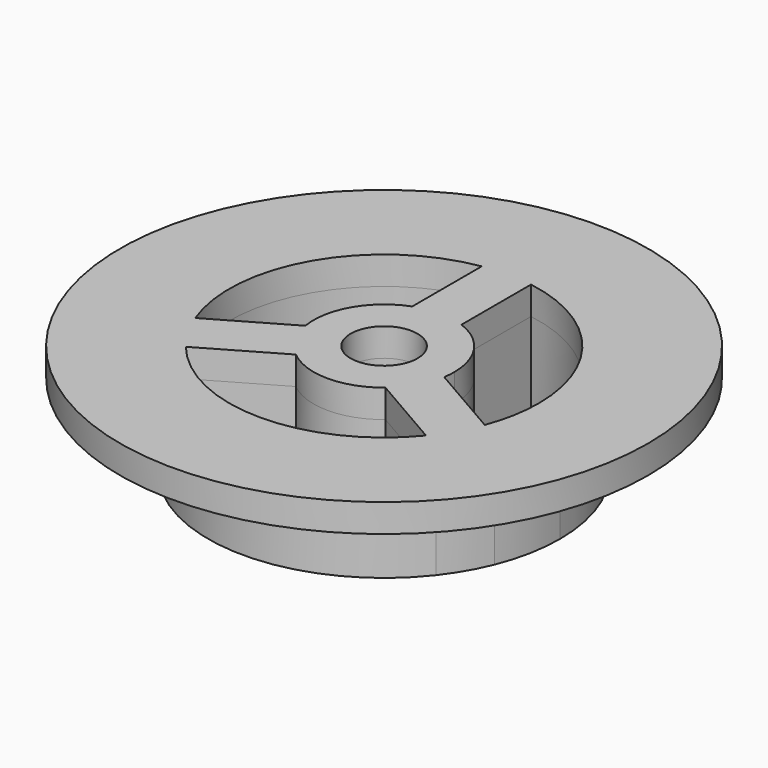
from build123d import *
from build123d import SkipClean  # not in build123d's __all__

# Parameters (mm, degrees)
F0_R     = 37.5
F0_R_2   = 4.75
F1_DEPTH = 4
F2_DEPTH = 12


with BuildPart() as f1:
    # F0 (on Top) → F1 (new body)
    with BuildSketch(Plane.XY):
        Circle(F0_R)
        with BuildLine():
            ThreePointArc((3.5, 24.753787589), (18.8745860882, 16.3935963108), (25, 0))
            ThreePointArc((25, 0), (24.5426691937, -4.7599778204), (23.1874088919, -9.3458048812))
            ThreePointArc((23.1874088919, -9.3458048812), (21.6506350946, -12.5), (19.6874088919, -15.4079827077))
            ThreePointArc((19.6874088919, -15.4079827077), (0, -25), (-19.6874088919, -15.4079827077))
            ThreePointArc((-19.6874088919, -15.4079827077), (-21.6506350946, -12.5), (-23.1874088919, -9.3458048812))
            ThreePointArc((-23.1874088919, -9.3458048812), (-21.6506350946, 12.5), (-3.5, 24.753787589))
            ThreePointArc((-3.5, 24.753787589), (0, 25), (3.5, 24.753787589))
        make_face(mode=Mode.SUBTRACT)
        with BuildLine():
            Line((3.5, 21.719806629), (3.5, 24.753787589))
            ThreePointArc((3.5, 24.753787589), (0, 25), (-3.5, 24.753787589))
            Line((-3.5, 24.753787589), (-3.5, 21.719806629))
            ThreePointArc((-3.5, 21.719806629), (0, 22), (3.5, 21.719806629))
        make_face()
        with BuildLine():
            Line((3.5, 9.3674969976), (3.5, 21.719806629))
            ThreePointArc((3.5, 21.719806629), (0, 22), (-3.5, 21.719806629))
            Line((-3.5, 21.719806629), (-3.5, 9.3674969976))
            ThreePointArc((-3.5, 9.3674969976), (0, 10), (3.5, 9.3674969976))
        make_face()
        with BuildLine():
            ThreePointArc((17.059904306, -13.8909922277), (19.0525588833, -11), (20.559904306, -7.8288144012))
            Line((20.559904306, -7.8288144012), (9.8624903698, -1.6526595856))
            ThreePointArc((9.8624903698, -1.6526595856), (8.6602540378, -5), (6.3624903698, -7.714837412))
            Line((6.3624903698, -7.714837412), (17.059904306, -13.8909922277))
        make_face()
        with BuildLine():
            ThreePointArc((19.6874088919, -15.4079827077), (21.6506350946, -12.5), (23.1874088919, -9.3458048812))
            Line((23.1874088919, -9.3458048812), (20.559904306, -7.8288144012))
            ThreePointArc((20.559904306, -7.8288144012), (19.0525588833, -11), (17.059904306, -13.8909922277))
            Line((17.059904306, -13.8909922277), (19.6874088919, -15.4079827077))
        make_face()
        with BuildLine():
            Line((-9.8624903698, -1.6526595856), (-20.559904306, -7.8288144012))
            ThreePointArc((-20.559904306, -7.8288144012), (-19.0525588833, -11), (-17.059904306, -13.8909922277))
            Line((-17.059904306, -13.8909922277), (-6.3624903698, -7.714837412))
            ThreePointArc((-6.3624903698, -7.714837412), (-8.6602540378, -5), (-9.8624903698, -1.6526595856))
        make_face()
        with BuildLine():
            Line((-20.559904306, -7.8288144012), (-23.1874088919, -9.3458048812))
            ThreePointArc((-23.1874088919, -9.3458048812), (-21.6506350946, -12.5), (-19.6874088919, -15.4079827077))
            Line((-19.6874088919, -15.4079827077), (-17.059904306, -13.8909922277))
            ThreePointArc((-17.059904306, -13.8909922277), (-19.0525588833, -11), (-20.559904306, -7.8288144012))
        make_face()
        with BuildLine():
            ThreePointArc((10, 0), (8.2158383626, 5.7008771255), (3.5, 9.3674969976))
            ThreePointArc((3.5, 9.3674969976), (0, 10), (-3.5, 9.3674969976))
            ThreePointArc((-3.5, 9.3674969976), (-8.6602540378, 5), (-9.8624903698, -1.6526595856))
            ThreePointArc((-9.8624903698, -1.6526595856), (-8.6602540378, -5), (-6.3624903698, -7.714837412))
            ThreePointArc((-6.3624903698, -7.714837412), (0, -10), (6.3624903698, -7.714837412))
            ThreePointArc((6.3624903698, -7.714837412), (8.6602540378, -5), (9.8624903698, -1.6526595856))
            ThreePointArc((9.8624903698, -1.6526595856), (9.9655632981, -0.8291852332), (10, 0))
        make_face()
        Circle(F0_R_2, mode=Mode.SUBTRACT)
        with BuildLine():
            ThreePointArc((23.1874088919, -9.3458048812), (24.5426691937, -4.7599778204), (25, 0))
            ThreePointArc((25, 0), (18.8745860882, 16.3935963108), (3.5, 24.753787589))
            Line((3.5, 24.753787589), (3.5, 21.719806629))
            ThreePointArc((3.5, 21.719806629), (16.7481342244, 14.2653426177), (22, 0))
            ThreePointArc((22, 0), (21.6369810132, -3.9800819884), (20.559904306, -7.8288144012))
            Line((20.559904306, -7.8288144012), (23.1874088919, -9.3458048812))
        make_face()
        with BuildLine():
            ThreePointArc((-19.6874088919, -15.4079827077), (0, -25), (19.6874088919, -15.4079827077))
            Line((19.6874088919, -15.4079827077), (17.059904306, -13.8909922277))
            ThreePointArc((17.059904306, -13.8909922277), (0, -22), (-17.059904306, -13.8909922277))
            Line((-17.059904306, -13.8909922277), (-19.6874088919, -15.4079827077))
        make_face()
        with BuildLine():
            Line((-3.5, 21.719806629), (-3.5, 24.753787589))
            ThreePointArc((-3.5, 24.753787589), (-21.6506350946, 12.5), (-23.1874088919, -9.3458048812))
            Line((-23.1874088919, -9.3458048812), (-20.559904306, -7.8288144012))
            ThreePointArc((-20.559904306, -7.8288144012), (-19.0525588833, 11), (-3.5, 21.719806629))
        make_face()
    extrude(amount=F1_DEPTH)

    # F0 (on Top) → F2 (join)
    with BuildSketch(Plane.XY):
        with BuildLine():
            ThreePointArc((23.1874088919, -9.3458048812), (24.5426691937, -4.7599778204), (25, 0))
            ThreePointArc((25, 0), (18.8745860882, 16.3935963108), (3.5, 24.753787589))
            Line((3.5, 24.753787589), (3.5, 21.719806629))
            ThreePointArc((3.5, 21.719806629), (16.7481342244, 14.2653426177), (22, 0))
            ThreePointArc((22, 0), (21.6369810132, -3.9800819884), (20.559904306, -7.8288144012))
            Line((20.559904306, -7.8288144012), (23.1874088919, -9.3458048812))
        make_face()
        with BuildLine():
            Line((3.5, 21.719806629), (3.5, 24.753787589))
            ThreePointArc((3.5, 24.753787589), (0, 25), (-3.5, 24.753787589))
            Line((-3.5, 24.753787589), (-3.5, 21.719806629))
            ThreePointArc((-3.5, 21.719806629), (0, 22), (3.5, 21.719806629))
        make_face()
        with BuildLine():
            Line((-3.5, 21.719806629), (-3.5, 24.753787589))
            ThreePointArc((-3.5, 24.753787589), (-21.6506350946, 12.5), (-23.1874088919, -9.3458048812))
            Line((-23.1874088919, -9.3458048812), (-20.559904306, -7.8288144012))
            ThreePointArc((-20.559904306, -7.8288144012), (-19.0525588833, 11), (-3.5, 21.719806629))
        make_face()
        with BuildLine():
            Line((-20.559904306, -7.8288144012), (-23.1874088919, -9.3458048812))
            ThreePointArc((-23.1874088919, -9.3458048812), (-21.6506350946, -12.5), (-19.6874088919, -15.4079827077))
            Line((-19.6874088919, -15.4079827077), (-17.059904306, -13.8909922277))
            ThreePointArc((-17.059904306, -13.8909922277), (-19.0525588833, -11), (-20.559904306, -7.8288144012))
        make_face()
        with BuildLine():
            ThreePointArc((-19.6874088919, -15.4079827077), (0, -25), (19.6874088919, -15.4079827077))
            Line((19.6874088919, -15.4079827077), (17.059904306, -13.8909922277))
            ThreePointArc((17.059904306, -13.8909922277), (0, -22), (-17.059904306, -13.8909922277))
            Line((-17.059904306, -13.8909922277), (-19.6874088919, -15.4079827077))
        make_face()
        with BuildLine():
            ThreePointArc((19.6874088919, -15.4079827077), (21.6506350946, -12.5), (23.1874088919, -9.3458048812))
            Line((23.1874088919, -9.3458048812), (20.559904306, -7.8288144012))
            ThreePointArc((20.559904306, -7.8288144012), (19.0525588833, -11), (17.059904306, -13.8909922277))
            Line((17.059904306, -13.8909922277), (19.6874088919, -15.4079827077))
        make_face()
        with BuildLine():
            Line((3.5, 9.3674969976), (3.5, 21.719806629))
            ThreePointArc((3.5, 21.719806629), (0, 22), (-3.5, 21.719806629))
            Line((-3.5, 21.719806629), (-3.5, 9.3674969976))
            ThreePointArc((-3.5, 9.3674969976), (0, 10), (3.5, 9.3674969976))
        make_face()
        with BuildLine():
            ThreePointArc((17.059904306, -13.8909922277), (19.0525588833, -11), (20.559904306, -7.8288144012))
            Line((20.559904306, -7.8288144012), (9.8624903698, -1.6526595856))
            ThreePointArc((9.8624903698, -1.6526595856), (8.6602540378, -5), (6.3624903698, -7.714837412))
            Line((6.3624903698, -7.714837412), (17.059904306, -13.8909922277))
        make_face()
        with BuildLine():
            Line((-9.8624903698, -1.6526595856), (-20.559904306, -7.8288144012))
            ThreePointArc((-20.559904306, -7.8288144012), (-19.0525588833, -11), (-17.059904306, -13.8909922277))
            Line((-17.059904306, -13.8909922277), (-6.3624903698, -7.714837412))
            ThreePointArc((-6.3624903698, -7.714837412), (-8.6602540378, -5), (-9.8624903698, -1.6526595856))
        make_face()
        with BuildLine():
            ThreePointArc((10, 0), (8.2158383626, 5.7008771255), (3.5, 9.3674969976))
            ThreePointArc((3.5, 9.3674969976), (0, 10), (-3.5, 9.3674969976))
            ThreePointArc((-3.5, 9.3674969976), (-8.6602540378, 5), (-9.8624903698, -1.6526595856))
            ThreePointArc((-9.8624903698, -1.6526595856), (-8.6602540378, -5), (-6.3624903698, -7.714837412))
            ThreePointArc((-6.3624903698, -7.714837412), (0, -10), (6.3624903698, -7.714837412))
            ThreePointArc((6.3624903698, -7.714837412), (8.6602540378, -5), (9.8624903698, -1.6526595856))
            ThreePointArc((9.8624903698, -1.6526595856), (9.9655632981, -0.8291852332), (10, 0))
        make_face()
        Circle(F0_R_2, mode=Mode.SUBTRACT)
    with SkipClean():  # cleaning this boolean's faces spoils the solid; the shape is the same uncleaned
        extrude(amount=-F2_DEPTH)


solid = f1.part
